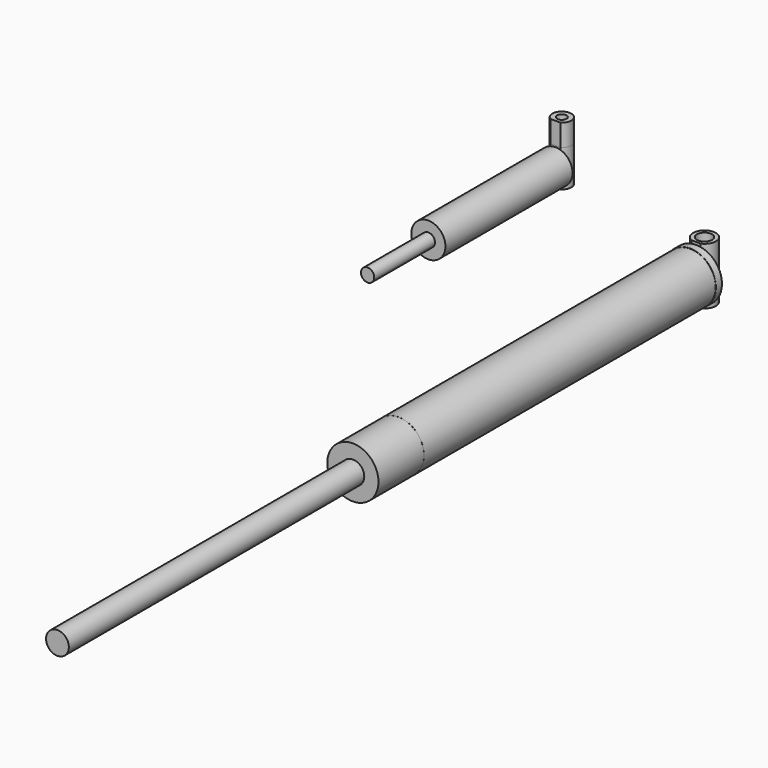
from build123d import *

# Parameters (mm, degrees)
F0_R          = 85.725
F0_R_2        = 76.2
F1_DEPTH      = 1219.2
F2_R          = 85.5895184233
F2_R_2        = 76.2
F2_R_3        = 38.1
F3_DEPTH      = 190.5
F4_R          = 86.3833911662
F4_R_2        = 85.725
F4_R_3        = 76.2
F5_DEPTH      = 25.4
F6_R          = 25.4
F7_DEPTH      = 95.25
F8_R          = 38.1
F9_DEPTH      = 1235.075
F9_DEPTH_BACK = 203.2
F16_R         = 15.875
F17_DEPTH     = 123.825
F18_DEPTH     = 73.025
F20_DEPTH     = 531.368
F21_R         = 57.15
F22_DEPTH     = 6.35
F23_R         = 56.7654297604
F24_DEPTH     = 6.35
F25_R         = 22.225
F26_DEPTH     = 254


with BuildPart() as f1:
    # F0 (on Front) → F1 (new body)
    with BuildSketch(Plane.XZ):
        Circle(F0_R)
        Circle(F0_R_2, mode=Mode.SUBTRACT)
    extrude(amount=F1_DEPTH)

    # F2 (on face) → F3 (join)
    with BuildSketch(Plane.XZ.offset(1219.2)):
        Circle(F2_R)
        Circle(F2_R_2, mode=Mode.SUBTRACT)
        Circle(F2_R_2)
        Circle(F2_R_3, mode=Mode.SUBTRACT)
    extrude(amount=F3_DEPTH)

    # F4 (on face) → F5 (join)
    with BuildSketch(Plane(origin=(0, 0, 0), x_dir=(-1, 0, 0), z_dir=(0, 1, 0))):
        Circle(F4_R)
        Circle(F4_R_2, mode=Mode.SUBTRACT)
        Circle(F4_R_2)
        Circle(F4_R_3, mode=Mode.SUBTRACT)
        Circle(F4_R_3)
    extrude(amount=F5_DEPTH)


with BuildPart() as f7:
    # F6 (on Top) → F7 (new body, symmetric)
    with BuildSketch(Plane.XY):
        with BuildLine():
            Line((-15.2267650865, 25.4), (15.2267650865, 25.4))
            ThreePointArc((15.2267650865, 25.4), (0, 98.425), (-15.2267650865, 25.4))
        make_face()
        with Locations((0, 60.325)):
            Circle(F6_R, mode=Mode.SUBTRACT)
    extrude(amount=F7_DEPTH, both=True)


with BuildPart() as f9:
    # F8 (on face) → F9 (new body, two sides)
    with BuildSketch(Plane.XZ.offset(1409.7)) as f9_sk:
        Circle(F8_R)
    extrude(amount=F9_DEPTH)
    extrude(f9_sk.sketch, amount=-F9_DEPTH_BACK)


with BuildPart() as f10_1:
    # F10: copy of F1
    add(f1.part.moved(Location((-444.5, 0, 0))))


with BuildPart() as f11_1:
    # F11: copy of F7
    add(f7.part.moved(Location((-347.98, 0, 0))))


with BuildPart() as f12_1:
    # F12: copy of F9
    add(f9.part.moved(Location((-424.18, 0, 0))))


with BuildPart() as f17:
    # F16 (on Top) → F17 (new body)
    with BuildSketch(Plane.XY):
        with BuildLine():
            Line((-610.2468481452, 178.5038380514), (-575.7917527592, 178.5038380514))
            ThreePointArc((-575.7917527592, 178.5038380514), (-593.0193004522, 236.9235605938), (-610.2468481452, 178.5038380514))
        make_face()
        with Locations((-593.0193004522, 205.1735605938)):
            Circle(F16_R, mode=Mode.SUBTRACT)
    extrude(amount=F17_DEPTH)


with BuildPart() as f18:
    # F18 (new): a face of the model
    f18_faces = [f17.part.faces().sort_by_distance(p)[0] for p in [
        (-593.0193004522, 179.3666887907, 123.825),
    ]]
    extrude(f18_faces, amount=F18_DEPTH)


with BuildPart() as f20:
    # F19 (on face) → F20 (new body)
    with BuildSketch(Plane.XZ.offset(-178.5038380514)):
        with BuildLine():
            ThreePointArc((-575.7917527592, 7.4209033957), (-546.9179075738, 28.1370048197), (-535.8693004522, 61.9125))
            ThreePointArc((-535.8693004522, 61.9125), (-546.9179075738, 95.6879951803), (-575.7917527592, 116.4040966043))
            Line((-575.7917527592, 116.4040966043), (-575.7917527592, 109.7021302809))
            ThreePointArc((-575.7917527592, 109.7021302809), (-551.4513073356, 91.1141970426), (-542.2193283862, 61.9125))
            ThreePointArc((-542.2193283862, 61.9125), (-551.4513073356, 32.7108029574), (-575.7917527592, 14.1228697191))
            Line((-575.7917527592, 14.1228697191), (-575.7917527592, 7.4209033957))
        make_face()
        with BuildLine():
            Line((-575.7917527592, 109.7021302809), (-575.7917527592, 116.4040966043))
            ThreePointArc((-575.7917527592, 116.4040966043), (-593.0193004522, 119.0625), (-610.2468481452, 116.4040966043))
            Line((-610.2468481452, 116.4040966043), (-610.2468481452, 109.7021302809))
            ThreePointArc((-610.2468481452, 109.7021302809), (-593.0193004522, 112.712472066), (-575.7917527592, 109.7021302809))
        make_face()
        with BuildLine():
            ThreePointArc((-610.2468481452, 7.4209033957), (-593.0193004522, 4.7625), (-575.7917527592, 7.4209033957))
            Line((-575.7917527592, 7.4209033957), (-575.7917527592, 14.1228697191))
            ThreePointArc((-575.7917527592, 14.1228697191), (-593.0193004522, 11.112527934), (-610.2468481452, 14.1228697191))
            Line((-610.2468481452, 14.1228697191), (-610.2468481452, 7.4209033957))
        make_face()
        with BuildLine():
            Line((-610.2468481452, 109.7021302809), (-610.2468481452, 116.4040966043))
            ThreePointArc((-610.2468481452, 116.4040966043), (-650.1693004522, 61.9125), (-610.2468481452, 7.4209033957))
            Line((-610.2468481452, 7.4209033957), (-610.2468481452, 14.1228697191))
            ThreePointArc((-610.2468481452, 14.1228697191), (-643.8192725182, 61.9125), (-610.2468481452, 109.7021302809))
        make_face()
    extrude(amount=F20_DEPTH)


with BuildPart() as f17_1:
    add(f17.part)

    add(f20.part)  # F22 merges F20
    # F21 (on face) → F22 (join)
    with BuildSketch(Plane(origin=(0, 178.5038380514, 0), x_dir=(-1, 0, 0), z_dir=(0, 1, 0))):
        with Locations((593.0193004522, 61.9125)):
            Circle(F21_R)
    extrude(amount=-F22_DEPTH)

    # F23 (on face) → F24 (join)
    with BuildSketch(Plane.XZ.offset(352.8641619486)):
        with Locations((-593.0193004522, 61.9125)):
            Circle(F23_R)
    extrude(amount=-F24_DEPTH)


with BuildPart() as f26:
    # F25 (on face) → F26 (new body, symmetric)
    with BuildSketch(Plane.XZ.offset(352.8641619486)):
        with Locations((-593.0193004522, 61.9125)):
            Circle(F25_R)
    extrude(amount=F26_DEPTH, both=True)


with BuildPart() as f17_2:
    add(f17_1.part)

    # F27: cut F26
    add(f26.part, mode=Mode.SUBTRACT)


solid = Compound([f1.part, f7.part, f9.part, f18.part, f26.part, f17_2.part])
